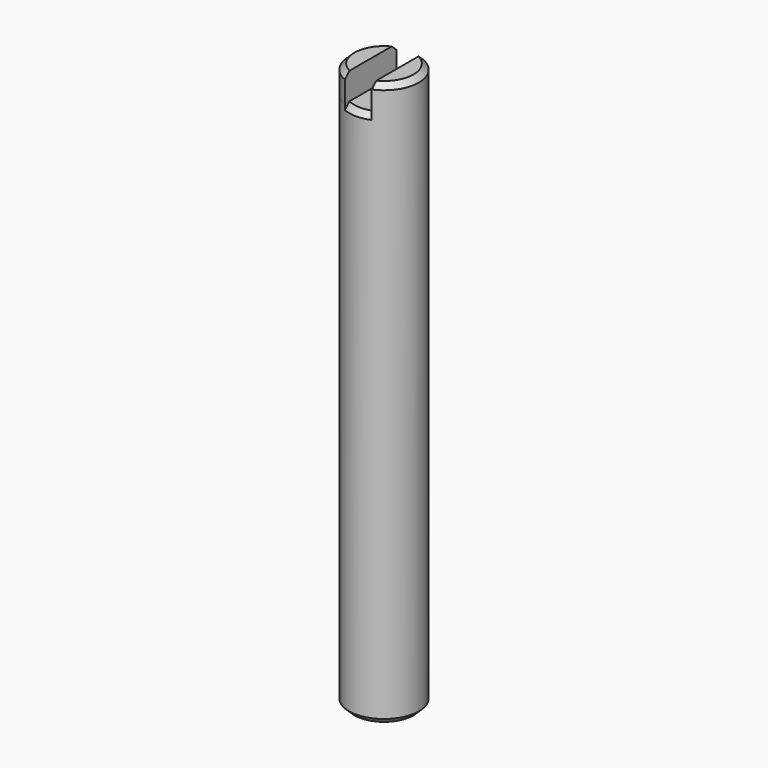
from build123d import *

# Parameters (mm, degrees)
F1_DEPTH     = 100
F2_DEPTH     = 5
F3_T2_ANGLE  = 180.1385265573
F3_T4_ANGLE  = 180.1385265573
F3_T10_ANGLE = 90.5817403508
F3_T16_ANGLE = 90.5817403508


# Not quite as in the source:
# - a fillet or chamfer that OpenCascade refuses, or shapes differently, is made with other operations: its cross-section is extruded or revolved along the edge and cut away or added


with BuildPart() as f1:
    # F0 (on Top) → F1 (new body)
    with BuildSketch(Plane.XY):
        with BuildLine():
            Line((-2.5, -6), (-2.5, 6))
            ThreePointArc((-2.5, 6), (-6.5, 0), (-2.5, -6))
        make_face()
        with BuildLine():
            ThreePointArc((2.5, -6), (5.4083269132, -3.6055512755), (6.5, 0))
            ThreePointArc((6.5, 0), (5.4083269132, 3.6055512755), (2.5, 6))
            Line((2.5, 6), (2.5, -6))
        make_face()
        with BuildLine():
            Line((2.5, -6), (2.5, 6))
            ThreePointArc((2.5, 6), (0, 6.5), (-2.5, 6))
            Line((-2.5, 6), (-2.5, -6))
            ThreePointArc((-2.5, -6), (0, -6.5), (2.5, -6))
        make_face()
    extrude(amount=-F1_DEPTH)

    # F0 (on Top) → F2 (join)
    with BuildSketch(Plane.XY):
        with BuildLine():
            Line((-2.5, -6), (-2.5, 6))
            ThreePointArc((-2.5, 6), (-6.5, 0), (-2.5, -6))
        make_face()
        with BuildLine():
            ThreePointArc((2.5, -6), (5.4083269132, -3.6055512755), (6.5, 0))
            ThreePointArc((6.5, 0), (5.4083269132, 3.6055512755), (2.5, 6))
            Line((2.5, 6), (2.5, -6))
        make_face()
    extrude(amount=F2_DEPTH)

    # F3: chamfer of 1 on 7 edges, made by hand

    # F3_s1 → F3_t2 (revolve, cut)
    with BuildSketch(Plane(origin=(0, 0, 0), x_dir=(0, 0, 1), z_dir=(0.9999992693, -0.001208872, 0))):
        Polygon((4, -6.5), (5, -5.5), (5, -6.5), align=None)
    revolve(axis=Axis((0, 0, 5), (0, 0, 1)), revolution_arc=F3_T2_ANGLE, mode=Mode.SUBTRACT)

    # F3_s3 → F3_t4 (revolve, cut)
    with BuildSketch(Plane(origin=(0, 0, 0), x_dir=(0, 0, 1), z_dir=(-0.9999992693, 0.001208872, 0))):
        Polygon((4, -6.5), (5, -5.5), (5, -6.5), align=None)
    revolve(axis=Axis((0, 0, 5), (0, 0, 1)), revolution_arc=F3_T4_ANGLE, mode=Mode.SUBTRACT)

    # F3_s5 → F3_t6 (revolve, cut)
    with BuildSketch(Plane(origin=(0, 0, 0), x_dir=(0, 0, 1), z_dir=(-0.9230769231, 0.3846153846, 0))):
        Polygon((-99, -6.5), (-100, -5.5), (-100, -6.5), align=None)
    revolve(axis=Axis((0, 0, -100), (0, 0, 1)), mode=Mode.SUBTRACT)


with BuildPart() as f3_tool8:
    # F3_s9 → F3_t10 (revolve)
    with BuildSketch(Plane(origin=(0, 0, 0), x_dir=(0, 0, 1), z_dir=(-0.7035079566, 0.7106873821, 0))):
        Polygon((-1, -6.5), (0, -5.5), (0, -6.5), align=None)
    revolve(axis=Axis((0, 0, 0), (0, 0, 1)), revolution_arc=F3_T10_ANGLE)

    split(bisect_by=Plane.YZ.offset(-2.5), keep=Keep.TOP)

    split(bisect_by=Plane.YZ.offset(2.5), keep=Keep.BOTTOM)


with BuildPart() as f1_1:
    add(f1.part)

    # F3_t7: cut F3_tool8
    add(f3_tool8.part, mode=Mode.SUBTRACT)


with BuildPart() as f3_tool14:
    # F3_s15 → F3_t16 (revolve)
    with BuildSketch(Plane(origin=(0, 0, 0), x_dir=(0, 0, 1), z_dir=(0.7035079566, -0.7106873821, 0))):
        Polygon((-1, -6.5), (0, -5.5), (0, -6.5), align=None)
    revolve(axis=Axis((0, 0, 0), (0, 0, 1)), revolution_arc=F3_T16_ANGLE)

    split(bisect_by=Plane.YZ.offset(-2.5), keep=Keep.TOP)

    split(bisect_by=Plane.YZ.offset(2.5), keep=Keep.BOTTOM)


with BuildPart() as f1_2:
    add(f1_1.part)

    # F3_t13: cut F3_tool14
    add(f3_tool14.part, mode=Mode.SUBTRACT)


solid = f1_2.part
